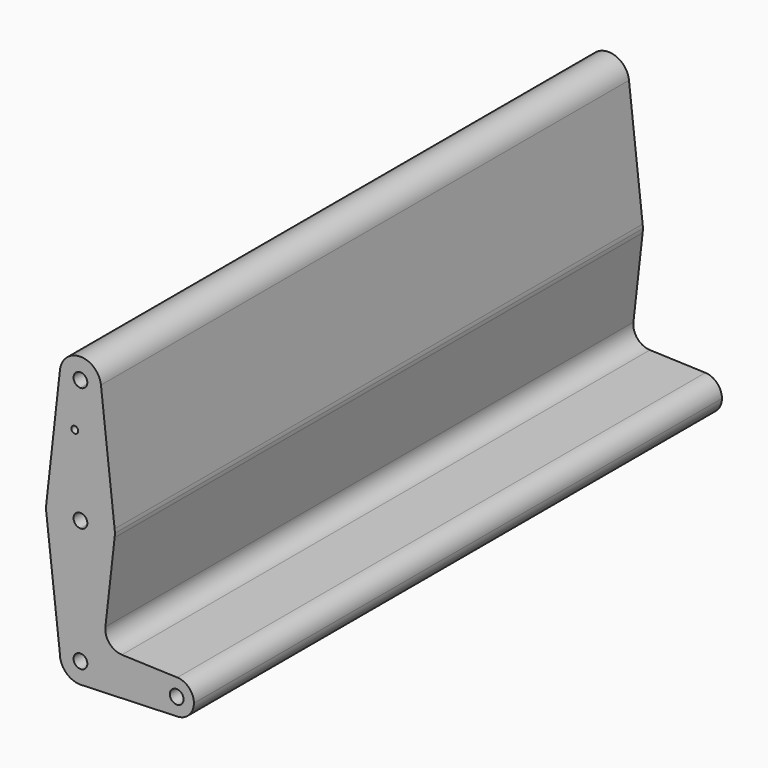
from build123d import *

# Parameters (mm, degrees)
F0_R     = 1.5875
F1_DEPTH = 304.8


# Not quite as in the source:
# - ends of sketch curves that miss each other by under 0.0002 mm in the source are joined


with BuildPart() as f1:
    # F0 (on Front) → F1 (new body)
    with BuildSketch(Plane.XZ):
        with BuildLine():
            Line((0, -35.9251248209), (0, -42.2751248896))
            ThreePointArc((0, -42.2751248896), (2.2450640303, -43.2050608593), (3.175, -45.4501248896))
            Line((3.175, -45.4501248896), (9.5250000687, -45.4501248896))
            ThreePointArc((9.5250000687, -45.4501248896), (6.7351921394, -38.7149327502), (0, -35.9251248209))
        make_face()
        with BuildLine():
            ThreePointArc((3.175, -45.4501248896), (-2.2450640303, -47.6951889199), (0, -42.2751248896))
            Line((0, -42.2751248896), (0, -35.9251248209))
            ThreePointArc((0, -35.9251248209), (-6.6836697304, -38.6638014929), (-9.5238937406, -45.3049548981))
            ThreePointArc((-9.5238937406, -45.3049548981), (-6.7863233967, -52.13379462), (0, -54.9751249583))
            Line((0, -54.9751249583), (0.6773435819, -54.951010742))
            ThreePointArc((0.6773435819, -54.951010742), (6.9705567917, -51.941424014), (9.5250000687, -45.4501248896))
            Line((9.5250000687, -45.4501248896), (3.175, -45.4501248896))
        make_face()
        with BuildLine():
            Line((36.5125, -45.4501248896), (9.5250000687, -45.4501248896))
            ThreePointArc((9.5250000687, -45.4501248896), (6.9705567917, -51.941424014), (0.6773435819, -54.951010742))
            Line((0.6773435819, -54.951010742), (44.7324052867, -53.3825995038))
            ThreePointArc((44.7324052867, -53.3825995038), (38.9380895197, -51.1617576778), (36.5125, -45.4501248896))
        make_face()
        with BuildLine():
            Line((0, -4.1751248896), (0, -35.9251248209))
            ThreePointArc((0, -35.9251248209), (6.7351921394, -38.7149327502), (9.5250000687, -45.4501248896))
            Line((9.5250000687, -45.4501248896), (36.5125, -45.4501248896))
            ThreePointArc((36.5125, -45.4501248896), (38.9380895197, -39.7384921015), (44.7324052867, -37.5176502755))
            Line((44.7324052867, -37.5176502755), (19.1378694473, -36.6064551461))
            ThreePointArc((19.1378694473, -36.6064551461), (13.3988872221, -33.8519658653), (11.5206935861, -27.7695718592))
            Line((11.5206935861, -27.7695718592), (15.7748262706, 9.9192906189))
            ThreePointArc((15.7748262706, 9.9192906189), (10.5770706294, -0.1382498214), (0, -4.1751248896))
        make_face()
        with BuildLine():
            ThreePointArc((-9.5238937406, -45.3049548981), (-6.6836697304, -38.6638014929), (0, -35.9251248209))
            Line((0, -35.9251248209), (0, -4.1751248896))
            ThreePointArc((0, -4.1751248896), (-10.5752191937, -0.1399037729), (-15.7742685853, 9.9143568106))
            Line((-15.7742685853, 9.9143568106), (-9.5238937406, -45.3049548981))
        make_face()
        with BuildLine():
            ThreePointArc((-15.7038062969, 14.0249757078), (-10.370743778, 23.7191637121), (0, 27.5748751104))
            Line((0, 27.5748751104), (0, 47.8104427457))
            Line((0, 47.8104427457), (0, 59.3248751104))
            ThreePointArc((0, 59.3248751104), (-7.0846213328, 62.4832617586), (-9.4708755422, 69.8638482188))
            Line((-9.4708755422, 69.8638482188), (-15.7038062969, 14.0249757078))
        make_face()
        with Locations((-2.6159647387, 47.8104427457)):
            Circle(F0_R, mode=Mode.SUBTRACT)
        with BuildLine():
            Line((0, 47.8104427457), (0, 27.5748751104))
            ThreePointArc((0, 27.5748751104), (10.5770706294, 23.5380000422), (15.7748262706, 13.4804596019))
            Line((15.7748262706, 13.4804596019), (9.4660212705, 69.9082069616))
            ThreePointArc((9.4660212705, 69.9082069616), (9.5102438875, 69.3798620908), (9.525, 68.8498751104))
            ThreePointArc((9.525, 68.8498751104), (6.7351920908, 62.1146830196), (0, 59.3248751104))
            Line((0, 59.3248751104), (0, 47.8104427457))
        make_face()
        with BuildLine():
            ThreePointArc((9.4660212705, 69.9082069616), (-0.0223117795, 78.3748489783), (-9.4708755422, 69.8638482188))
            ThreePointArc((-9.4708755422, 69.8638482188), (-7.0846213328, 62.4832617586), (0, 59.3248751104))
            ThreePointArc((0, 59.3248751104), (6.7351920908, 62.1146830196), (9.525, 68.8498751104))
            ThreePointArc((9.525, 68.8498751104), (9.5102438875, 69.3798620908), (9.4660212705, 69.9082069616))
        make_face()
        with BuildLine():
            ThreePointArc((3.175, 68.8498751104), (2.2450640303, 66.6048110801), (0, 65.6748751104))
            ThreePointArc((0, 65.6748751104), (-2.2450640303, 71.0949391407), (3.175, 68.8498751104))
        make_face(mode=Mode.SUBTRACT)
        with BuildLine():
            ThreePointArc((44.7324052867, -37.5176502755), (38.9380895197, -39.7384921015), (36.5125, -45.4501248896))
            ThreePointArc((36.5125, -45.4501248896), (38.9380895197, -51.1617576778), (44.7324052867, -53.3825995038))
            ThreePointArc((44.7324052867, -53.3825995038), (50.1616327882, -50.96203537), (52.3875, -45.4501248896))
            ThreePointArc((52.3875, -45.4501248896), (50.1616327882, -39.9382144093), (44.7324052867, -37.5176502755))
        make_face()
        with BuildLine():
            ThreePointArc((47.625, -45.4501248896), (44.45, -48.6251248896), (41.275, -45.4501248896))
            ThreePointArc((41.275, -45.4501248896), (44.45, -42.2751248896), (47.625, -45.4501248896))
        make_face(mode=Mode.SUBTRACT)
        with BuildLine():
            Line((0, 8.5248751104), (0, -4.1751248896))
            ThreePointArc((0, -4.1751248896), (10.5770706294, -0.1382498214), (15.7748262706, 9.9192906189))
            ThreePointArc((15.7748262706, 9.9192906189), (15.8499367829, 10.8081750617), (15.875, 11.6998751104))
            ThreePointArc((15.875, 11.6998751104), (15.8499367829, 12.5915751591), (15.7748262706, 13.4804596019))
            ThreePointArc((15.7748262706, 13.4804596019), (10.5770706294, 23.5380000422), (0, 27.5748751104))
            Line((0, 27.5748751104), (0, 14.8748751104))
            ThreePointArc((0, 14.8748751104), (2.2450640303, 13.9449391407), (3.175, 11.6998751104))
            ThreePointArc((3.175, 11.6998751104), (2.2450640303, 9.4548110801), (0, 8.5248751104))
        make_face()
        with BuildLine():
            ThreePointArc((-15.7742685853, 9.9143568106), (-10.5752191937, -0.1399037729), (0, -4.1751248896))
            Line((0, -4.1751248896), (0, 8.5248751104))
            ThreePointArc((0, 8.5248751104), (-3.175, 11.6998751104), (0, 14.8748751104))
            Line((0, 14.8748751104), (0, 27.5748751104))
            ThreePointArc((0, 27.5748751104), (-10.370743778, 23.7191637121), (-15.7038062969, 14.0249757078))
            Line((-15.7038062969, 14.0249757078), (-15.8299773584, 12.8946310826))
            ThreePointArc((-15.8299773584, 12.8946310826), (-15.8722272886, 11.4031835217), (-15.7742685853, 9.9143568106))
        make_face()
    extrude(amount=F1_DEPTH)


solid = f1.part
